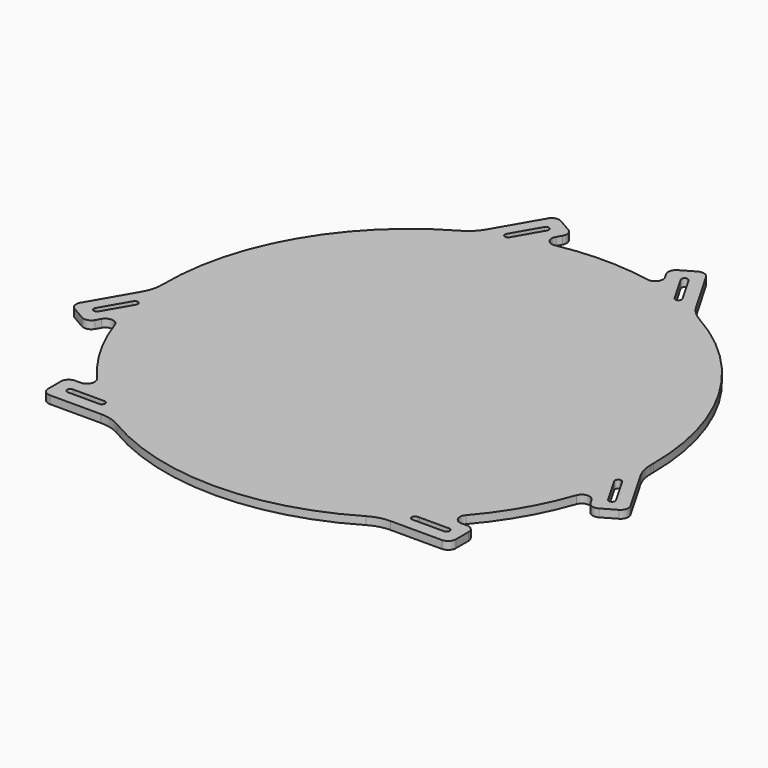
from build123d import *

# Parameters (mm, degrees)
F1_DEPTH = 5
F2_R     = 5
F3_R     = 5
F4_R     = 25


# Not quite as in the source:
# - ends of sketch curves that miss each other by under 0.0002 mm in the source are joined


with BuildPart() as f1:
    # F0 (on Top) → F1 (new body)
    with BuildSketch(Plane.XY):
        with BuildLine():
            ThreePointArc((154.7685858954, -8.4666888412), (154.9421356729, -4.2349253955), (155, 0))
            ThreePointArc((155, 0), (132.0663621555, 81.1386220428), (70.0519227484, 138.2668728194))
            ThreePointArc((70.0519227484, 138.2668728194), (62.8960752724, 141.6653934994), (55.5759359282, 144.6938676852))
            ThreePointArc((55.5759359282, 144.6938676852), (53.8706420703, 143.993176318), (52.3166727987, 144.9852322827))
            Line((52.3166727987, 144.9852322827), (51.6490211362, 146.1416388839))
            ThreePointArc((51.6490211362, 146.1416388839), (46.0520817915, 148.0006951425), (40.3884712615, 149.6454856959))
            ThreePointArc((40.3884712615, 149.6454856959), (2.3057e-06, 155), (-40.3884668093, 149.6454868975))
            ThreePointArc((-40.3884668093, 149.6454868975), (-46.0520770675, 148.0006966124), (-51.6490161547, 146.1416406444))
            Line((-51.6490161547, 146.1416406445), (-52.3166688853, 144.9852321932))
            ThreePointArc((-52.3166688853, 144.9852321932), (-53.8706389409, 143.9931761584), (-55.5759330313, 144.6938687979))
            ThreePointArc((-55.5759330313, 144.6938687979), (-62.8960721537, 141.665394884), (-70.0519194288, 138.2668745012))
            ThreePointArc((-70.0519194288, 138.2668745012), (-134.2339375866, 77.5), (-154.7685855343, -8.4666954414))
            ThreePointArc((-154.7685855343, -8.4666954414), (-154.1338668835, -16.3631011587), (-153.0965326665, -24.2167645548))
            ThreePointArc((-153.0965326665, -24.2167645548), (-151.9167610651, -24.9023775772), (-151.4512795032, -26.1850518006))
            ThreePointArc((-151.4512795032, -26.1850518006), (-151.5194278506, -26.7026898908), (-151.7192286956, -27.1850518006))
            Line((-151.7192286956, -27.1850518006), (-152.3868814262, -28.3414602518))
            ThreePointArc((-152.3868814262, -28.3414602518), (-151.1984015779, -34.1180796687), (-149.7910266196, -39.845305172))
            ThreePointArc((-149.7910266196, -39.845305172), (-134.2339373892, -77.500000342), (-109.4025592509, -109.8001822829))
            ThreePointArc((-109.4025592509, -109.8001822829), (-105.1463222254, -113.8826190535), (-100.7378611443, -117.800183922))
            Line((-100.7378611443, -117.8001839221), (-99.4025592509, -117.8001839221))
            ThreePointArc((-99.4025592509, -117.8001839221), (-97.9883456885, -118.3859703597), (-97.4025592509, -119.8001839221))
            ThreePointArc((-97.4025592509, -119.8001839221), (-97.4322899717, -120.143751918), (-97.5205982187, -120.4771053897))
            ThreePointArc((-97.5205982187, -120.4771053897), (-91.2377891853, -125.3022977626), (-84.7166561444, -129.8001855612))
            ThreePointArc((-84.7166561444, -129.8001855612), (0, -155), (84.7166561444, -129.8001855612))
            ThreePointArc((84.7166561444, -129.8001855612), (91.2377891853, -125.3022977626), (97.5205982187, -120.4771053897))
            ThreePointArc((97.5205982187, -120.4771053897), (97.7664292231, -118.6499324137), (99.4025592509, -117.8001839221))
            Line((99.4025592509, -117.8001839221), (100.7378611443, -117.8001839221))
            ThreePointArc((100.7378611443, -117.800183922), (105.1463222254, -113.8826190535), (109.4025592509, -109.8001822829))
            ThreePointArc((109.4025592509, -109.8001822829), (134.233938542, -77.4999983451), (149.791027805, -39.8453007155))
            ThreePointArc((149.791027805, -39.8453007155), (151.1984026669, -34.1180748426), (152.3868823923, -28.3414550574))
            Line((152.3868823923, -28.3414550574), (151.719230036, -27.1850472546))
            ThreePointArc((151.719230036, -27.1850472546), (151.6370691989, -25.3432419871), (153.0965333673, -24.2167601241))
            ThreePointArc((153.0965333673, -24.2167601241), (154.1338674692, -16.3630956418), (154.7685858954, -8.4666888412))
        make_face()
        with BuildLine():
            ThreePointArc((55.5759359282, 144.6938676852), (62.8960752724, 141.6653934994), (70.0519227484, 138.2668728194))
            Line((70.0519227484, 138.2668728194), (47.7089766448, 176.9659938193))
            Line((47.7089766448, 176.9659938193), (30.3884705677, 166.9659949732))
            Line((30.3884705677, 166.9659949732), (40.3884712615, 149.6454856959))
            ThreePointArc((40.3884712615, 149.6454856959), (46.0520817915, 148.0006951425), (51.6490211362, 146.1416388839))
            Line((51.6490211362, 146.1416388839), (42.3166727987, 162.3057403584))
            ThreePointArc((42.3166727987, 162.3057403584), (43.0487236063, 165.037791166), (45.7807744138, 164.3057403584))
            Line((45.7807744138, 164.3057403584), (55.7807744138, 146.9852322827))
            ThreePointArc((55.7807744138, 146.9852322827), (55.9805752588, 146.5028703729), (56.0487236063, 145.9852322827))
            ThreePointArc((56.0487236063, 145.9852322827), (55.9268110169, 145.2976367053), (55.5759359282, 144.6938676852))
        make_face()
        with BuildLine():
            Line((177.1115338821, -47.1658099451), (154.7685858954, -8.4666888412))
            ThreePointArc((154.7685858954, -8.4666888412), (154.1338674692, -16.3630956418), (153.0965333673, -24.2167601241))
            ThreePointArc((153.0965333673, -24.2167601241), (154.2930861111, -24.3708356099), (155.1833316512, -25.1850472546))
            Line((155.1833316512, -25.1850472546), (165.1833316512, -42.5055553303))
            ThreePointArc((165.1833316512, -42.5055553303), (165.3831324962, -42.9879172401), (165.4512808436, -43.5055553303))
            ThreePointArc((165.4512808436, -43.5055553303), (163.9689189338, -45.4374069829), (161.719230036, -44.5055553303))
            Line((161.719230036, -44.5055553303), (152.3868823923, -28.3414550574))
            ThreePointArc((152.3868823923, -28.3414550574), (151.1984026669, -34.1180748426), (149.791027805, -39.8453007155))
            Line((149.791027805, -39.8453007155), (159.791027805, -57.1658087912))
            Line((159.791027805, -57.1658087912), (177.1115338821, -47.1658099451))
        make_face()
        with BuildLine():
            ThreePointArc((-51.6490161547, 146.1416406444), (-46.0520770675, 148.0006966124), (-40.3884668093, 149.6454868975))
            Line((-40.3884668093, 149.6454868975), (-30.3884668093, 166.9659949732))
            Line((-30.3884668093, 166.9659949732), (-47.7089725764, 176.9659936403))
            Line((-47.7089725764, 176.9659936403), (-70.0519194288, 138.2668745012))
            ThreePointArc((-70.0519194288, 138.2668745012), (-62.8960721537, 141.665394884), (-55.5759330313, 144.6938687979))
            ThreePointArc((-55.5759330313, 144.6938687979), (-56.0407757277, 145.8071514412), (-55.7807705004, 146.9852321932))
            Line((-55.7807705004, 146.9852321932), (-45.7807705004, 164.3057402689))
            ThreePointArc((-45.7807705004, 164.3057402689), (-43.5310816027, 165.2375919215), (-42.0487196929, 163.3057402689))
            ThreePointArc((-42.0487196929, 163.3057402689), (-42.1168680403, 162.7881021787), (-42.3166688853, 162.3057402689))
            Line((-42.3166688853, 162.3057402689), (-51.6490161547, 146.1416406445))
        make_face()
        with BuildLine():
            Line((129.4025592509, -109.8001822829), (109.4025592509, -109.8001822829))
            ThreePointArc((109.4025592509, -109.8001822829), (105.1463222254, -113.8826190535), (100.7378611443, -117.800183922))
            Line((100.7378611443, -117.800183922), (119.4025592509, -117.8001839221))
            ThreePointArc((119.4025592509, -117.8001839221), (120.8167728132, -118.3859703597), (121.4025592509, -119.8001839221))
            ThreePointArc((121.4025592509, -119.8001839221), (120.8167728132, -121.2143974844), (119.4025592509, -121.8001839221))
            Line((119.4025592509, -121.8001839221), (99.4025592509, -121.8001842499))
            ThreePointArc((99.4025592509, -121.8001842499), (98.2523077425, -121.4363139498), (97.5205982187, -120.4771053897))
            ThreePointArc((97.5205982187, -120.4771053897), (91.2377891853, -125.3022977626), (84.7166561444, -129.8001855612))
            Line((84.7166561444, -129.8001855612), (129.4025592509, -129.8001855612))
            Line((129.4025592509, -129.8001855612), (129.4025592509, -109.8001822829))
        make_face()
        with BuildLine():
            ThreePointArc((-153.0965326665, -24.2167645548), (-154.1338668835, -16.3631011587), (-154.7685855343, -8.4666954414))
            Line((-154.7685855343, -8.4666954414), (-177.1115323867, -47.1658145805))
            Line((-177.1115323867, -47.1658145805), (-159.7910266196, -57.1658132477))
            Line((-159.7910266196, -57.1658132477), (-149.7910266196, -39.845305172))
            ThreePointArc((-149.7910266196, -39.845305172), (-151.1984015779, -34.1180796687), (-152.3868814262, -28.3414602518))
            Line((-152.3868814262, -28.3414602518), (-161.7192286956, -44.5055598762))
            ThreePointArc((-161.7192286956, -44.5055598762), (-164.4512795032, -45.2376106838), (-165.1833303107, -42.5055598762))
            Line((-165.1833303107, -42.5055598762), (-155.1833303107, -25.1850518006))
            ThreePointArc((-155.1833303107, -25.1850518006), (-154.2930850654, -24.3708402927), (-153.0965326665, -24.2167645548))
        make_face()
        with BuildLine():
            Line((-129.4025592509, -129.8001855612), (-84.7166561444, -129.8001855612))
            ThreePointArc((-84.7166561444, -129.8001855612), (-91.2377891853, -125.3022977626), (-97.5205982187, -120.4771053897))
            ThreePointArc((-97.5205982187, -120.4771053897), (-98.2523077425, -121.4363139498), (-99.4025592509, -121.8001839221))
            Line((-99.4025592509, -121.8001839221), (-119.4025592509, -121.8001839221))
            ThreePointArc((-119.4025592509, -121.8001839221), (-121.4025592509, -119.8001839221), (-119.4025592509, -117.8001839221))
            Line((-119.4025592509, -117.8001839221), (-100.7378611443, -117.8001839221))
            ThreePointArc((-100.7378611443, -117.800183922), (-105.1463222254, -113.8826190535), (-109.4025592509, -109.8001822829))
            Line((-109.4025592509, -109.8001822829), (-129.4025592509, -109.8001822829))
            Line((-129.4025592509, -109.8001822829), (-129.4025592509, -129.8001855612))
        make_face()
    extrude(amount=F1_DEPTH)

    # F2
    f2_edges = [f1.edges().sort_by_distance(p)[0] for p in [
        (-47.708973, 176.965994, 2.5),
        (-30.388467, 166.965995, 2.5),
        (30.388471, 166.965995, 2.5),
        (47.708977, 176.965994, 2.5),
        (177.111534, -47.16581, 2.5),
        (-177.111532, -47.165815, 2.5),
        (-129.402559, -109.800182, 2.5),
        (129.402559, -109.800182, 2.5),
        (159.791028, -57.165809, 2.5),
        (129.402559, -129.800186, 2.5),
        (-129.402559, -129.800186, 2.5),
        (-159.791027, -57.165813, 2.5),
    ]]
    fillet(f2_edges, radius=F2_R)

    # F3
    f3_edges = [f1.edges().sort_by_distance(p)[0] for p in [
        (-149.791027, -39.845305, 2.5),
        (149.791028, -39.845301, 2.5),
        (40.388471, 149.645486, 2.5),
        (-40.388467, 149.645487, 2.5),
        (-109.402559, -109.800182, 2.5),
        (109.402559, -109.800182, 2.5),
    ]]
    fillet(f3_edges, radius=F3_R)

    # F4
    f4_edges = [f1.edges().sort_by_distance(p)[0] for p in [
        (-70.051919, 138.266875, 2.5),
        (-154.768586, -8.466695, 2.5),
        (70.051923, 138.266873, 2.5),
        (154.768586, -8.466689, 2.5),
        (-84.716656, -129.800186, 2.5),
        (84.716656, -129.800186, 2.5),
    ]]
    fillet(f4_edges, radius=F4_R)


solid = f1.part
